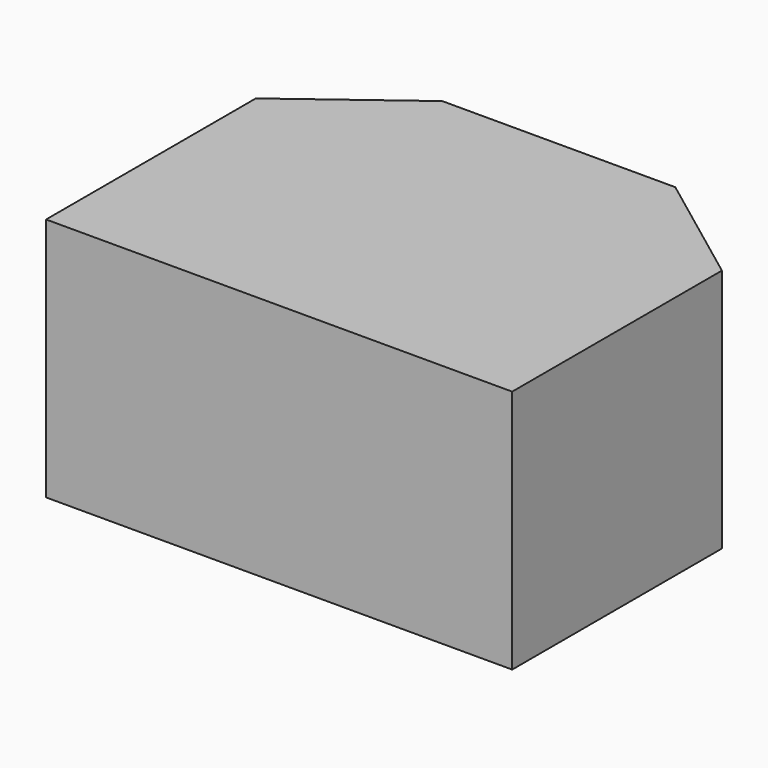
from build123d import *

# Parameters (mm, degrees)
F0_W     = 1500
F0_H     = 1500
F1_DEPTH = 2100
F2_W     = 1671.5718507767
F2_H     = 758.528470993
F3_DEPTH = 25
F4_T     = -2.5


# Not quite as in the source:
# - a shell that OpenCascade refuses in one call is made with other operations: the cavity is built on its own and cut out


with BuildPart() as f1:
    # F0 (on Top) → F1 (new body)
    with BuildSketch(Plane.XY):
        with Locations((-1250, -750)):
            Rectangle(F0_W, F0_H)
        Polygon((2000, 750), (-2000, 750), (-2000, 0), (-500, 0), (-500, -1500), (2000, -1500), align=None)
        Polygon((1000, 1500), (-1000, 1500), (-2000, 750), (2000, 750), align=None)
    extrude(amount=F1_DEPTH)

    # F2 (on face) → F3 (cut)
    with BuildSketch(Plane(origin=(0, 1500, 0), x_dir=(-1, 0, 0), z_dir=(0, 1, 0))):
        with Locations((0, 1529.2642354965)):
            Rectangle(F2_W, F2_H)
    extrude(amount=-F3_DEPTH, mode=Mode.SUBTRACT)

    # F4: a shell. OpenCascade refuses it in one call, so the cavity is built on its own and cut out:
    # the body offset inwards by the wall thickness, plus a prism from it out through each open face.
    f4_core = offset(f1.part, amount=F4_T, kind=Kind.INTERSECTION, mode=Mode.PRIVATE)
    f4_exits = [f4_core.faces().sort_by_distance(p)[0] for p in [
        (0, 1472.5, 1529.264235),
    ]]
    add(f4_core, mode=Mode.SUBTRACT)
    extrude(f4_exits, amount=-F4_T, mode=Mode.SUBTRACT)


solid = f1.part
